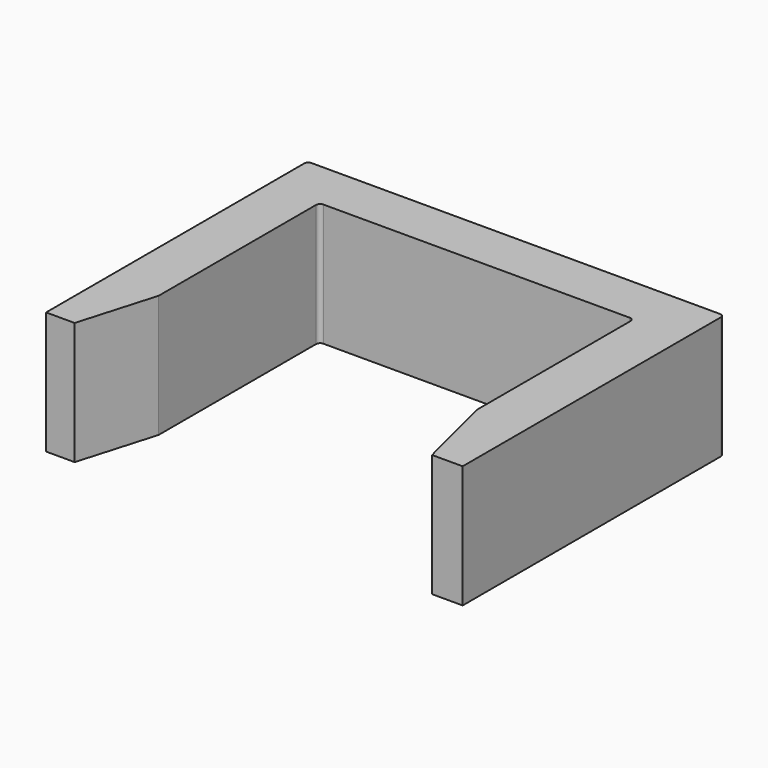
from build123d import *

# Parameters (mm, degrees)
F1_DEPTH    = 15
F2_R        = 0.5
F3_T1_DEPTH = 66.9437702684
F4_SIZE2    = 2.5
F4_SIZE     = 10


# Not quite as in the source:
# - a fillet or chamfer that OpenCascade refuses, or shapes differently, is made with other operations: its cross-section is extruded or revolved along the edge and cut away or added


with BuildPart() as f1:
    # F0 (on Top) → F1 (new body)
    with BuildSketch(Plane.XY):
        Polygon((25.5, 20), (-25.5, 20), (-25.5, -20), (-19.5, -20), (-19.25, -14), (-19.25, 14), (19.25, 14), (19.25, -14), (19.25, -20), (25.5, -20), align=None)
    extrude(amount=F1_DEPTH)

    # F2
    f2_edges = [f1.edges().sort_by_distance(p)[0] for p in [
        (-19.25, 14, 7.5),
        (19.25, 14, 7.5),
        (-25.5, 20, 7.5),
        (25.5, 20, 7.5),
    ]]
    fillet(f2_edges, radius=F2_R)

    # F3: chamfer of 10 x 2.5 on 1 edges, made by hand

    # F3_s2 → F3_t1 (cut)
    with BuildSketch(Plane.XY.offset(-25.9718851342)):
        Polygon((-22, -20), (-19.0836945529, -10.0086692691), (-19.5, -20), align=None)
    extrude(amount=F3_T1_DEPTH, mode=Mode.SUBTRACT)

    # F4
    f4_edges = [f1.edges().sort_by_distance(p)[0] for p in [
        (19.25, -20, 7.5),
    ]]
    f4_side = f1.faces().sort_by_distance((19.25, -3.25, 7.5))[0]
    chamfer(f4_edges, length=F4_SIZE, length2=F4_SIZE2, reference=f4_side)


solid = f1.part
